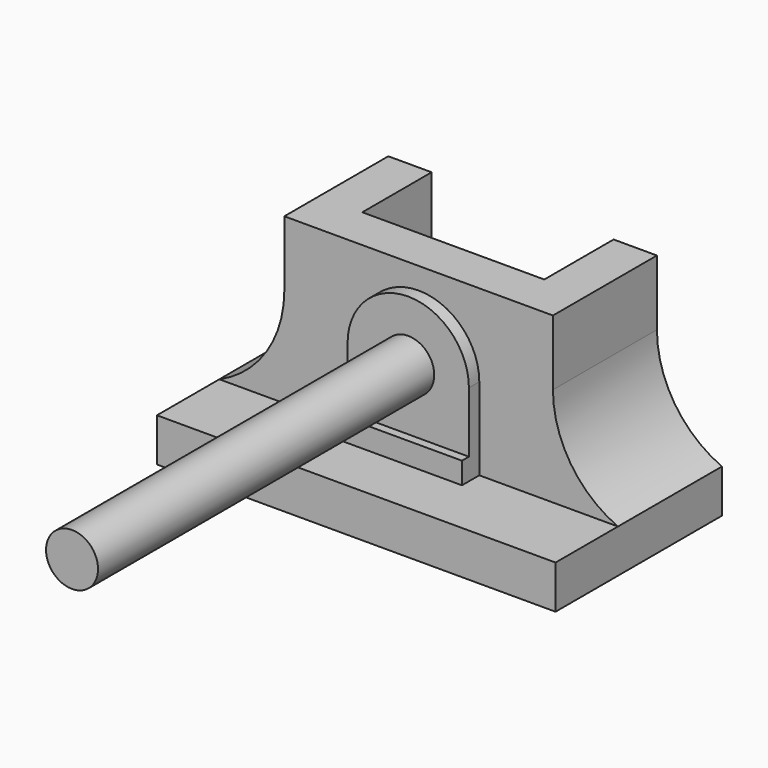
from build123d import *

# Parameters (mm, degrees)
F1_DEPTH    = 48
F0_W        = 92
F0_H        = 18
F2_DEPTH    = 10
F3_W        = 15
F3_H        = 38
F4_DEPTH    = 50
F5_T1_DEPTH = 30
F6_R        = 6
F7_DEPTH    = 3
F8_DEPTH    = 5
F9_DEPTH    = 25
F10_DEPTH   = 100


# Not quite as in the source:
# - a fillet or chamfer that OpenCascade refuses, or shapes differently, is made with other operations: its cross-section is extruded or revolved along the edge and cut away or added


with BuildPart() as f1:
    # F0 (on Top) → F1 (new body)
    with BuildSketch(Plane.XY):
        Polygon((-46, 30), (-46, 0), (46, 0), (46, 30), (21, 30), (21, 10), (-21, 10), (-21, 30), align=None)
    extrude(amount=F1_DEPTH)

    # F0 (on Top) → F2 (join)
    with BuildSketch(Plane.XY):
        with Locations((0, -9)):
            Rectangle(F0_W, F0_H)
    extrude(amount=F2_DEPTH)

    # F3 (on face) → F4 (cut)
    with BuildSketch(Plane.XZ):
        Polygon((-31, 48), (-31, 58.456501329), (-68.4553310275, 62.7410188317), (-62.9399716854, 10), (-46, 10), (-46, 48), align=None)
        with Locations((-38.5, 29)):
            Rectangle(F3_W, F3_H)
        with Locations((38.5, 29)):
            Rectangle(F3_W, F3_H)
        Polygon((31, 58.8478222489), (31, 48), (46, 48), (46, 10), (62.6155510545, 10), (62.6155510545, 62.4165832996), align=None)
    extrude(amount=-F4_DEPTH, mode=Mode.SUBTRACT)

    # F5: fillet of radius 25 on 2 edges, made by hand

    # F5_s2 → F5_t1 (join)
    with BuildSketch(Plane.XZ.offset(-30)):
        with BuildLine():
            ThreePointArc((-31, 32.9128784748), (-35.0834993366, 19.2198145372), (-46, 10))
            Line((-46, 10), (-31, 10))
            Line((-31, 10), (-31, 32.9128784748))
        make_face()
        with BuildLine():
            ThreePointArc((31, 32.9128784748), (35.0834993366, 19.2198145372), (46, 10))
            Line((46, 10), (31, 10))
            Line((31, 10), (31, 32.9128784748))
        make_face()
    extrude(amount=F5_T1_DEPTH)

    # F6 (on face) → F7 (join)
    with BuildSketch(Plane.XZ):
        with BuildLine():
            ThreePointArc((0, 15), (9.8994949366, 19.1005050634), (14, 29))
            ThreePointArc((14, 29), (0, 43), (-14, 29))
            ThreePointArc((-14, 29), (-9.8994949366, 19.1005050634), (0, 15))
        make_face()
        with Locations((0, 29)):
            Circle(F6_R, mode=Mode.SUBTRACT)
        with BuildLine():
            ThreePointArc((0, 15), (-9.8994949366, 19.1005050634), (-14, 29))
            Line((-14, 29), (-14, 15))
            Line((-14, 15), (0, 15))
        make_face()
        with BuildLine():
            Line((14, 15), (14, 29))
            ThreePointArc((14, 29), (9.8994949366, 19.1005050634), (0, 15))
            Line((0, 15), (14, 15))
        make_face()
    extrude(amount=F7_DEPTH)

    # F6 (on face) → F8 (join)
    with BuildSketch(Plane.XZ):
        Polygon((14, 15), (0, 15), (-14, 15), (-14, 10), (14, 10), align=None)
    extrude(amount=F8_DEPTH)

    # F6 (on face) → F9 (cut)
    with BuildSketch(Plane.XZ):
        with Locations((0, 29)):
            Circle(F6_R)
    extrude(amount=-F9_DEPTH, mode=Mode.SUBTRACT)


with BuildPart() as f10:
    # F6 (on face) → F10 (new body)
    with BuildSketch(Plane.XZ):
        with Locations((0, 29)):
            Circle(F6_R)
    extrude(amount=F10_DEPTH)


solid = Compound([f1.part, f10.part])
